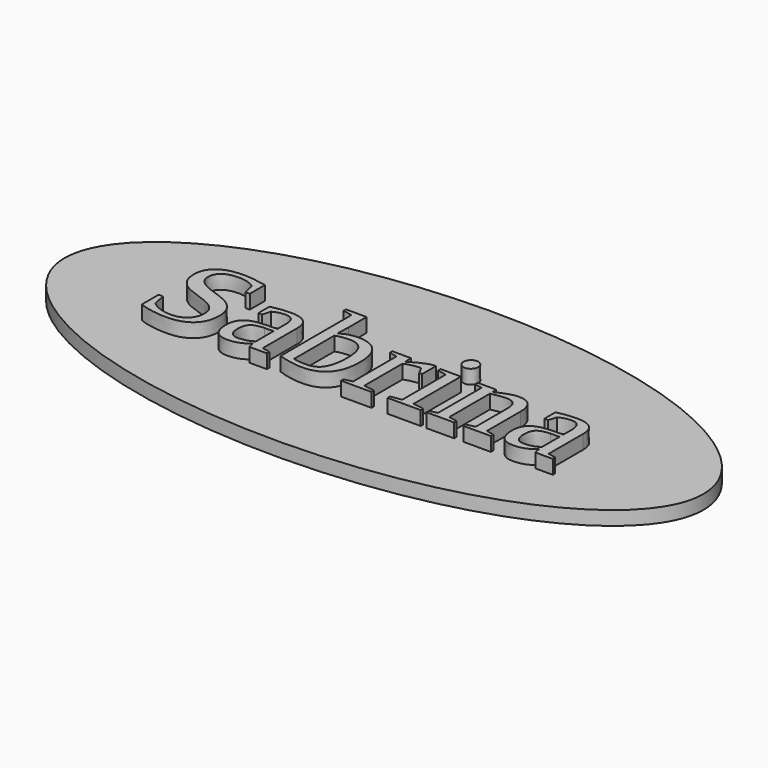
from build123d import *

# Parameters (mm, degrees)
F1_DEPTH     = 2.54
F2_TEXT_SIZE = 25.2518810293
F3_DEPTH     = 2.54


# Not quite as in the source:
# - Text() gives the source's letters only with a copy of the font that has no kerning and outlines rounded to 1/6400 em; it was checked with that copy


with BuildPart() as f1:
    # F0 (on Top) → F1 (new body)
    with BuildSketch(Plane.XY):
        with BuildLine():
            add(Edge.make_bspline(
                [(-57.9559616745, 0), (-57.9559616745, -43.3067268083), (28.9779808372, -21.6533634042), (115.9119233489, 0), (28.9779808372, 21.6533634042), (-57.9559616745, 43.3067268083), (-57.9559616745, 0)],
                knots=[0, 0, 0, 2.0943951024, 2.0943951024, 4.1887902048, 4.1887902048, 6.2831853072, 6.2831853072, 6.2831853072], degree=2, weights=[1, 0.5, 1, 0.5, 1, 0.5, 1]))
        make_face()
    extrude(amount=F1_DEPTH)

    # F2 (on face) → F3 (join)
    with BuildSketch(Plane.XY.offset(2.54)):
        with Locations((-39.1838172659, -8.728492782)):
            Text('Sabrina', F2_TEXT_SIZE, font='Tinos', text_align=(TextAlign.LEFT, TextAlign.BOTTOM))
    extrude(amount=F3_DEPTH)


solid = f1.part
